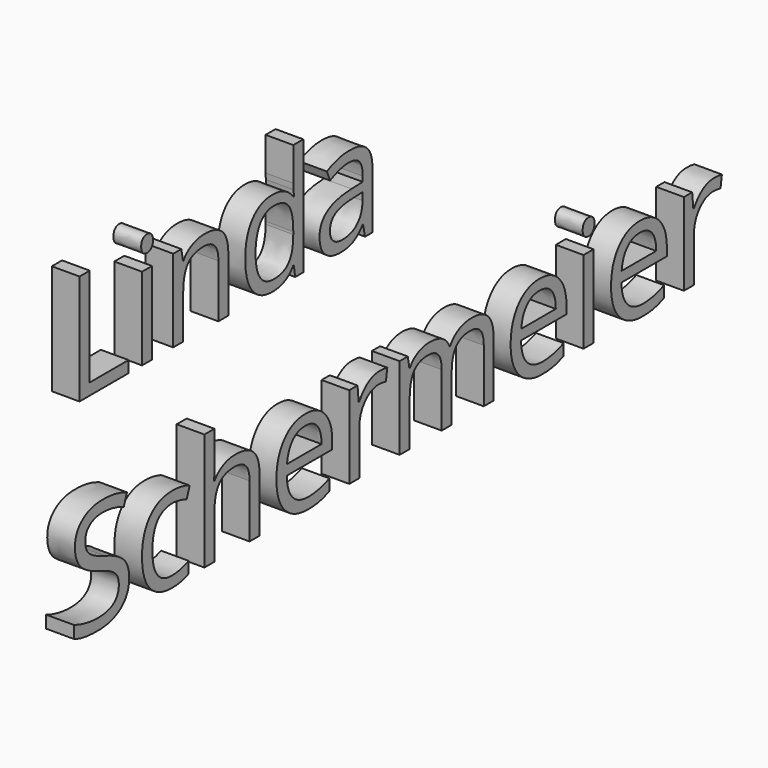
from build123d import *

# Parameters (mm, degrees)
F0_TEXT_SIZE = 141.3402561512
F1_DEPTH     = 25.4


# Not quite as in the source:
# - Text() gives the source's letters only with a copy of the font that has no kerning and outlines rounded to 1/6400 em; it was checked with that copy


with BuildPart() as f1:
    # F0 (on Right) → F1 (new body)
    with BuildSketch(Plane.YZ):
        with Locations((-379.6642208787, 0)):
            Text('Linda', F0_TEXT_SIZE, font='Open Sans', text_align=(TextAlign.LEFT, TextAlign.BOTTOM))
        with Locations((-379.6642208787, -192.2227483657)):
            Text('Schermeier', F0_TEXT_SIZE, font='Open Sans', text_align=(TextAlign.LEFT, TextAlign.BOTTOM))
    extrude(amount=F1_DEPTH)


solid = f1.part
